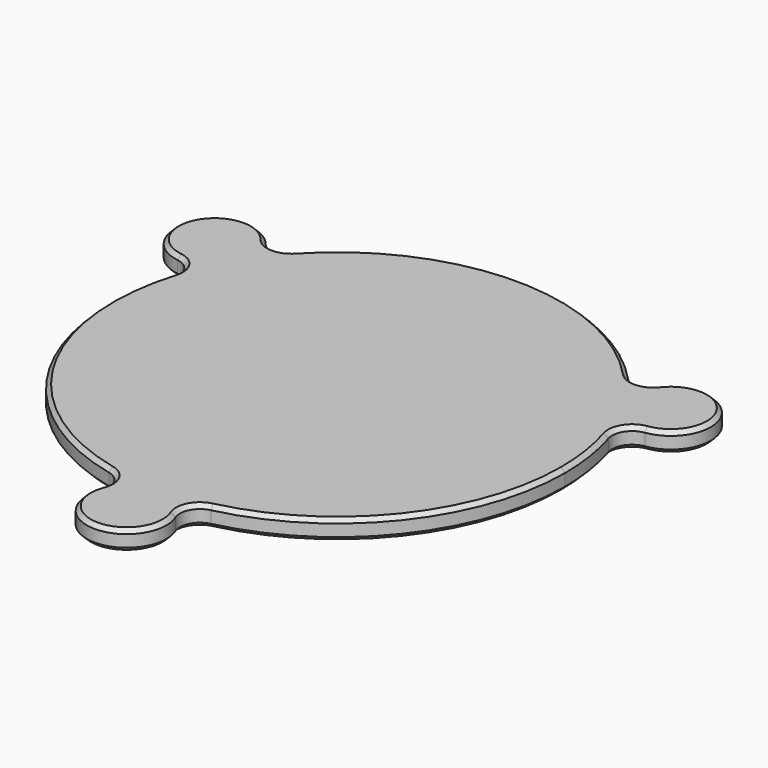
from build123d import *

# Parameters (mm, degrees)
F1_DEPTH = 5
F2_R     = 5
F3_SIZE  = 1


with BuildPart() as f1:
    # F0 (on Top) → F1 (new body)
    with BuildSketch(Plane.XY):
        with BuildLine():
            ThreePointArc((-51.3934756327, 24.996663025), (-49.4933518263, 28.575), (-47.3444830059, 32.0097239742))
            ThreePointArc((-47.3444830059, 32.0097239742), (-65.9478344982, 38.075), (-51.3934756327, 24.996663025))
        make_face()
        with BuildLine():
            ThreePointArc((47.3444830059, 32.0097239742), (49.4933518263, 28.575), (51.3934756327, 24.996663025))
            ThreePointArc((51.3934756327, 24.996663025), (65.9478344982, 38.075), (47.3444830059, 32.0097239742))
        make_face()
        with BuildLine():
            ThreePointArc((4.0489926269, -57.0063869992), (41.8181923846, -38.9533218826), (57.15, 0))
            ThreePointArc((57.15, 0), (55.6922778867, 12.8254701198), (51.3934756327, 24.996663025))
            ThreePointArc((51.3934756327, 24.996663025), (49.4933518263, 28.575), (47.3444830059, 32.0097239742))
            ThreePointArc((47.3444830059, 32.0097239742), (0, 57.15), (-47.3444830059, 32.0097239742))
            ThreePointArc((-47.3444830059, 32.0097239742), (-49.4933518263, 28.575), (-51.3934756327, 24.996663025))
            ThreePointArc((-51.3934756327, 24.996663025), (-49.4933518263, -28.575), (-4.0489926269, -57.0063869992))
            ThreePointArc((-4.0489926269, -57.0063869992), (0, -57.15), (4.0489926269, -57.0063869992))
        make_face()
        with BuildLine():
            ThreePointArc((-4.0489926269, -57.0063869992), (0, -76.15), (4.0489926269, -57.0063869992))
            ThreePointArc((4.0489926269, -57.0063869992), (0, -57.15), (-4.0489926269, -57.0063869992))
        make_face()
    extrude(amount=F1_DEPTH)

    # F2
    f2_edges = [f1.edges().sort_by_distance(p)[0] for p in [
        (-4.048993, -57.006387, 2.5),
        (-47.344483, 32.009724, 2.5),
        (51.393476, 24.996663, 2.5),
        (-51.393476, 24.996663, 2.5),
        (4.048993, -57.006387, 2.5),
        (47.344483, 32.009724, 2.5),
    ]]
    fillet(f2_edges, radius=F2_R)

    # F3
    f3_edges = [f1.edges().sort_by_distance(p)[0] for p in [
        (-65.947834, 38.075, 0),
        (-45.702262, 37.347671, 0),
        (-55.195163, 20.905484, 0),
        (0, 57.15, 0),
        (-49.493352, -28.575, 0),
        (45.702262, 37.347671, 0),
        (-9.492901, -58.253155, 0),
        (65.947834, 38.075, 0),
        (0, -76.15, 0),
        (55.195163, 20.905484, 0),
        (9.492901, -58.253155, 0),
        (49.493352, -28.575, 0),
        (-65.947834, 38.075, 5),
        (-45.702262, 37.347671, 5),
        (-55.195163, 20.905484, 5),
        (0, 57.15, 5),
        (-49.493352, -28.575, 5),
        (45.702262, 37.347671, 5),
        (-9.492901, -58.253155, 5),
        (65.947834, 38.075, 5),
        (0, -76.15, 5),
        (55.195163, 20.905484, 5),
        (9.492901, -58.253155, 5),
        (49.493352, -28.575, 5),
    ]]
    chamfer(f3_edges, length=F3_SIZE)


solid = f1.part
